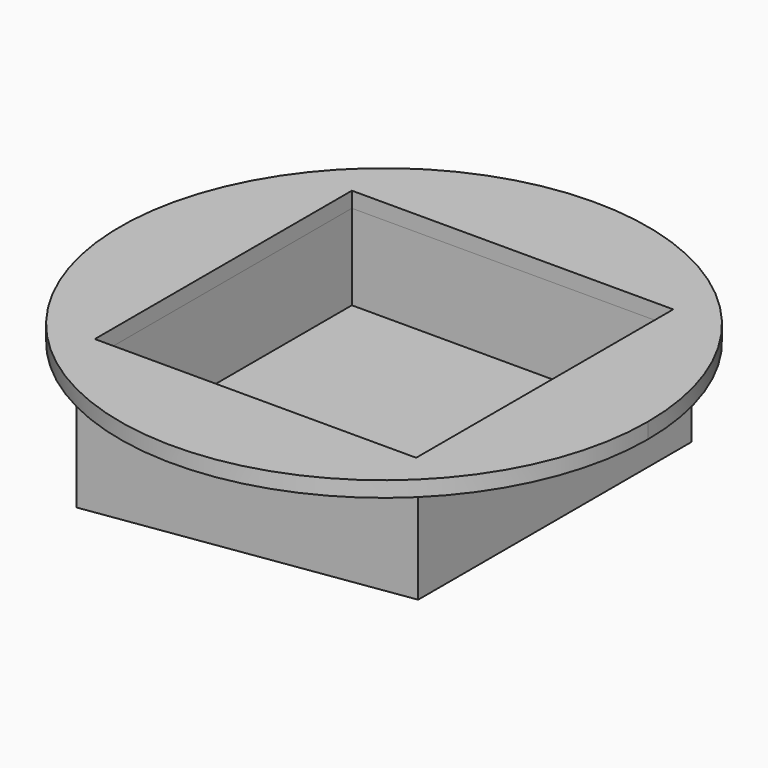
from build123d import *

# Parameters (mm, degrees)
F0_W     = 44
F0_H     = 44
F0_R     = 1.5
F1_DEPTH = 6
F2_W     = 44
F2_H     = 44
F2_W_2   = 41.4
F2_H_2   = 41.4
F3_DEPTH = 11
F4_W     = 44
F4_H     = 44
F5_DEPTH = 2
F7_DEPTH = 56.001


# Not quite as in the source:
# - the program builds the solid bodies; features that only make, move or delete a surface that nothing else refers to are left out


with BuildPart() as f1:
    # F0 (on Top) → F1 (new body)
    with BuildSketch(Plane.XY):
        Rectangle(F0_W, F0_H)
        with Locations((0, -17.25)):
            Circle(F0_R, mode=Mode.SUBTRACT)
        with Locations((-17.25, 0)):
            Circle(F0_R, mode=Mode.SUBTRACT)
        with Locations((17.25, 0)):
            Circle(F0_R, mode=Mode.SUBTRACT)
        with Locations((0, 17.25)):
            Circle(F0_R, mode=Mode.SUBTRACT)
        with Locations((0, -17.25)):
            Circle(F0_R)
        with Locations((-17.25, 0)):
            Circle(F0_R)
        with Locations((17.25, 0)):
            Circle(F0_R)
        with Locations((0, 17.25)):
            Circle(F0_R)
    extrude(amount=F1_DEPTH)

    # F2 (on face) → F3 (join)
    with BuildSketch(Plane.XY.offset(6)):
        Rectangle(F2_W, F2_H)
        Rectangle(F2_W_2, F2_H_2, mode=Mode.SUBTRACT)
    extrude(amount=F3_DEPTH)

    # F6 (on face) → F7 (cut, through all)
    with BuildSketch(Plane.XZ.offset(22)):
        Polygon((-22, 0), (22, 0), (22, 3.8495011951), align=None)
    extrude(amount=-F7_DEPTH, mode=Mode.SUBTRACT)


with BuildPart() as f5:
    # F4 (on face) → F5 (new body)
    with BuildSketch(Plane.XY.offset(17)):
        with BuildLine():
            ThreePointArc((34, 0), (31.4119041054, 13.0112367004), (24.0416305603, 24.0416305603))
            ThreePointArc((24.0416305603, 24.0416305603), (-31.4119041054, -13.0112367004), (34, 0))
        make_face()
        Rectangle(F4_W, F4_H, mode=Mode.SUBTRACT)
        Polygon((22, 22), (-22, 22), (-20.7, 20.7), (20.7, 20.7), align=None)
        Polygon((22, -22), (22, 22), (20.7, 20.7), (20.7, -20.7), align=None)
        Polygon((-20.7, 20.7), (-22, 22), (-22, -22), (-20.7, -20.7), align=None)
        Polygon((-20.7, -20.7), (-22, -22), (22, -22), (20.7, -20.7), align=None)
    extrude(amount=F5_DEPTH)


solid = Compound([f1.part, f5.part])
